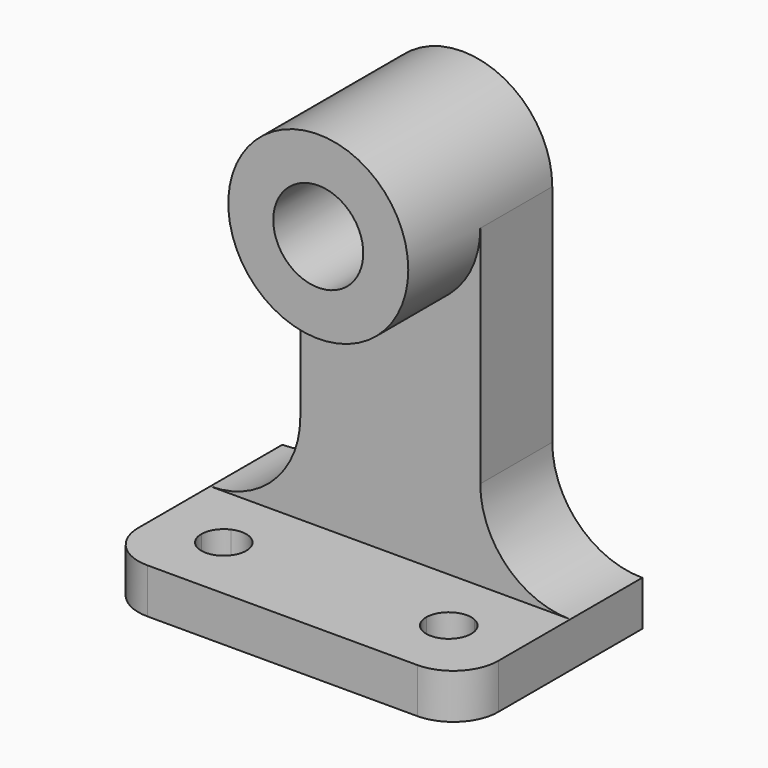
from build123d import *
from build123d import SkipClean  # not in build123d's __all__

# Parameters (mm, degrees)
F0_W     = 50.8
F0_H     = 6.35
F1_DEPTH = 31.75
F3_DEPTH = 19.05
F4_DEPTH = 6.35
F6_DEPTH = 6.351


with BuildPart() as f1:
    # F0 (on Front) → F1 (new body)
    with BuildSketch(Plane.XZ):
        with Locations((25.4, 3.175)):
            Rectangle(F0_W, F0_H)
        with BuildLine():
            ThreePointArc((12.7, 19.05), (8.9802561211, 10.0697438789), (0, 6.35))
            Line((0, 6.35), (50.8, 6.35))
            ThreePointArc((50.8, 6.35), (41.8197438789, 10.0697438789), (38.1, 19.05))
            Line((38.1, 19.05), (38.1, 50.8))
            ThreePointArc((38.1, 50.8), (25.4, 38.1), (12.7, 50.8))
            Line((12.7, 50.8), (12.7, 19.05))
        make_face()
        with BuildLine():
            Line((19.05, 50.8), (12.7, 50.8))
            ThreePointArc((12.7, 50.8), (25.4, 38.1), (38.1, 50.8))
            Line((38.1, 50.8), (31.75, 50.8))
            ThreePointArc((31.75, 50.8), (25.4, 44.45), (19.05, 50.8))
        make_face()
        with BuildLine():
            ThreePointArc((38.1, 50.8), (25.4, 63.5), (12.7, 50.8))
            Line((12.7, 50.8), (19.05, 50.8))
            ThreePointArc((19.05, 50.8), (25.4, 57.15), (31.75, 50.8))
            Line((31.75, 50.8), (38.1, 50.8))
        make_face()
    extrude(amount=-F1_DEPTH)

    # F2 (on face) → F3 (cut)
    with BuildSketch(Plane.XZ):
        with BuildLine():
            ThreePointArc((12.7, 19.05), (8.9802561211, 10.0697438789), (0, 6.35))
            Line((0, 6.35), (50.8, 6.35))
            ThreePointArc((50.8, 6.35), (41.8197438789, 10.0697438789), (38.1, 19.05))
            Line((38.1, 19.05), (38.1, 50.8))
            ThreePointArc((38.1, 50.8), (25.4, 38.1), (12.7, 50.8))
            Line((12.7, 50.8), (12.7, 19.05))
        make_face()
    with SkipClean():  # cleaning this boolean's faces spoils the solid; the shape is the same uncleaned
        extrude(amount=-F3_DEPTH, mode=Mode.SUBTRACT)

    # F4 (cut): a face of the model
    f4_faces = [f1.faces().sort_by_distance(p)[0] for p in [
        (25.4, 0, 63.1407897552),
    ]]
    extrude(f4_faces, amount=-F4_DEPTH, mode=Mode.SUBTRACT)

    # F5 (on face) → F6 (cut, through all)
    with BuildSketch(Plane.XY.offset(6.35)):
        with BuildLine():
            ThreePointArc((12.7, 9.525), (11.2473638622, 12.1922247236), (8.2186848968, 12.4188151032))
            ThreePointArc((8.2186848968, 12.4188151032), (10.3079286634, 11.3156118148), (11.849261314, 9.525))
            Line((11.849261314, 9.525), (12.7, 9.525))
        make_face()
        with BuildLine():
            ThreePointArc((11.849261314, 9.525), (10.3079286634, 11.3156118148), (8.2186848968, 12.4188151032))
            ThreePointArc((8.2186848968, 12.4188151032), (6.8577752764, 11.2473638622), (6.35, 9.525))
            Line((6.35, 9.525), (11.849261314, 9.525))
        make_face()
        with BuildLine():
            ThreePointArc((6.35, 9.525), (8.8568824776, 6.4210921444), (12.4188151032, 8.2186848968))
            ThreePointArc((12.4188151032, 8.2186848968), (12.1708000125, 8.8878706063), (11.849261314, 9.525))
            Line((11.849261314, 9.525), (6.35, 9.525))
        make_face()
        with BuildLine():
            ThreePointArc((11.849261314, 9.525), (12.1708000125, 8.8878706063), (12.4188151032, 8.2186848968))
            ThreePointArc((12.4188151032, 8.2186848968), (12.6289078556, 8.8568824776), (12.7, 9.525))
            Line((12.7, 9.525), (11.849261314, 9.525))
        make_face()
        with BuildLine():
            ThreePointArc((38.950738686, 9.525), (40.4920713366, 11.3156118148), (42.5813151032, 12.4188151032))
            ThreePointArc((42.5813151032, 12.4188151032), (39.5526361378, 12.1922247236), (38.1, 9.525))
            Line((38.1, 9.525), (38.950738686, 9.525))
        make_face()
        with BuildLine():
            ThreePointArc((44.45, 9.525), (43.9422247236, 11.2473638622), (42.5813151032, 12.4188151032))
            ThreePointArc((42.5813151032, 12.4188151032), (40.4920713366, 11.3156118148), (38.950738686, 9.525))
            Line((38.950738686, 9.525), (44.45, 9.525))
        make_face()
        with BuildLine():
            ThreePointArc((38.950738686, 9.525), (38.6291999875, 8.8878706063), (38.3811848968, 8.2186848968))
            ThreePointArc((38.3811848968, 8.2186848968), (41.9431175224, 6.4210921444), (44.45, 9.525))
            Line((44.45, 9.525), (38.950738686, 9.525))
        make_face()
        with BuildLine():
            ThreePointArc((38.1, 9.525), (38.1710921444, 8.8568824776), (38.3811848968, 8.2186848968))
            ThreePointArc((38.3811848968, 8.2186848968), (38.6291999875, 8.8878706063), (38.950738686, 9.525))
            Line((38.950738686, 9.525), (38.1, 9.525))
        make_face()
        with BuildLine():
            Line((44.45, 0), (50.8, 0))
            Line((50.8, 0), (50.8, 6.35))
            ThreePointArc((50.8, 6.35), (48.9401280605, 1.8598719395), (44.45, 0))
        make_face()
        with BuildLine():
            Line((0, 0), (6.35, 0))
            ThreePointArc((6.35, 0), (1.8598719395, 1.8598719395), (0, 6.35))
            Line((0, 6.35), (0, 0))
        make_face()
    extrude(amount=-F6_DEPTH, mode=Mode.SUBTRACT)


solid = f1.part
